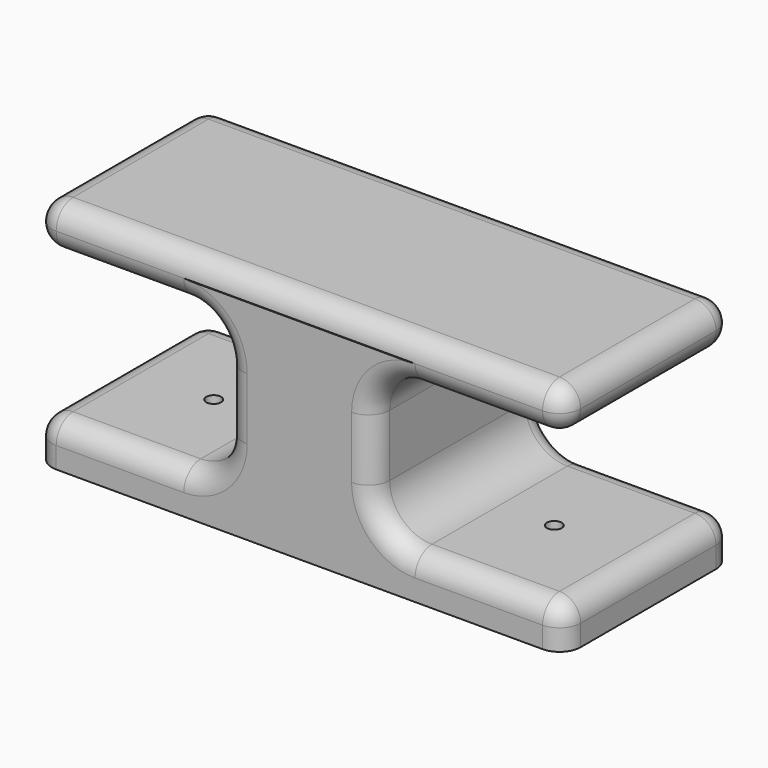
from build123d import *

# Parameters (mm, degrees)
F0_W     = 34.6808620631
F0_H     = 50
F1_DEPTH = 10
F2_DEPTH = 50
F3_W     = 125
F3_H     = 10
F4_DEPTH = 25
F5_R     = 10
F6_R     = 5
F7_R     = 5
F8_D     = 3.5
F8_DEPTH = 12
F8_TIP   = 1.0515060833
F9_R     = 4.99999


# Not quite as in the source:
# - a fillet or chamfer is up to 0.001 mm smaller than in the source, because OpenCascade refuses the exact size


with BuildPart() as f1:
    # F0 (on Top) → F1 (new body)
    with BuildSketch(Plane.XY):
        Polygon((-17.3404310315, -25), (-17.3404310315, 25), (-40.2640256677, 25), (-62.5, 25), (-62.5, -25), (-40.2640256677, -25), align=None)
        Polygon((62.5, -25), (62.5, 25), (40.2640256677, 25), (17.3404310315, 25), (17.3404310315, -25), (40.2640256677, -25), align=None)
        Rectangle(F0_W, F0_H)
    extrude(amount=F1_DEPTH)

    # F0 (on Top) → F2 (join)
    with BuildSketch(Plane.XY):
        Rectangle(F0_W, F0_H)
    extrude(amount=F2_DEPTH)

    # F3 (on Front) → F4 (join, symmetric)
    with BuildSketch(Plane.XZ):
        with Locations((0, 49.6251098812)):
            Rectangle(F3_W, F3_H)
    extrude(amount=F4_DEPTH, both=True)

    # F5
    f5_edges = [f1.edges().sort_by_distance(p)[0] for p in [
        (-17.340431, 0, 10),
        (17.340431, 0, 10),
        (17.340431, 0, 44.62511),
        (-17.340431, 0, 44.62511),
    ]]
    fillet(f5_edges, radius=F5_R)

    # F6
    f6_edges = [f1.edges().sort_by_distance(p)[0] for p in [
        (44.920216, -25, 10),
        (44.920216, 25, 10),
        (-44.920216, -25, 10),
        (-44.920216, 25, 10),
    ]]
    fillet(f6_edges, radius=F6_R)

    # F7
    f7_edges = [f1.edges().sort_by_distance(p)[0] for p in [
        (-62.5, 0, 10),
        (-62.5, 0, 44.62511),
        (62.5, 0, 10),
        (62.5, 0, 44.62511),
    ]]
    fillet(f7_edges, radius=F7_R)

    # F8
    with Locations(Plane(origin=(0, 0, 0), x_dir=(1, 0, 0), z_dir=(0, 0, -1))):
        with Locations((-40.2640256677, 0), (40.2640256677, 0)):
            Hole(F8_D / 2, depth=F8_DEPTH)
            with Locations((0, 0, -(F8_DEPTH + F8_TIP / 2))):  # 118° drill point
                Cone(0, F8_D / 2, F8_TIP, mode=Mode.SUBTRACT)

    # F9 (radius 5 in the source; OpenCascade refuses exactly that, so slightly less here)
    f9_edges = [f1.edges().sort_by_distance(p)[0] for p in [
        (0, 25, 54.62511),
        (62.5, 0, 54.62511),
    ]]
    fillet(f9_edges, radius=F9_R)


solid = f1.part
